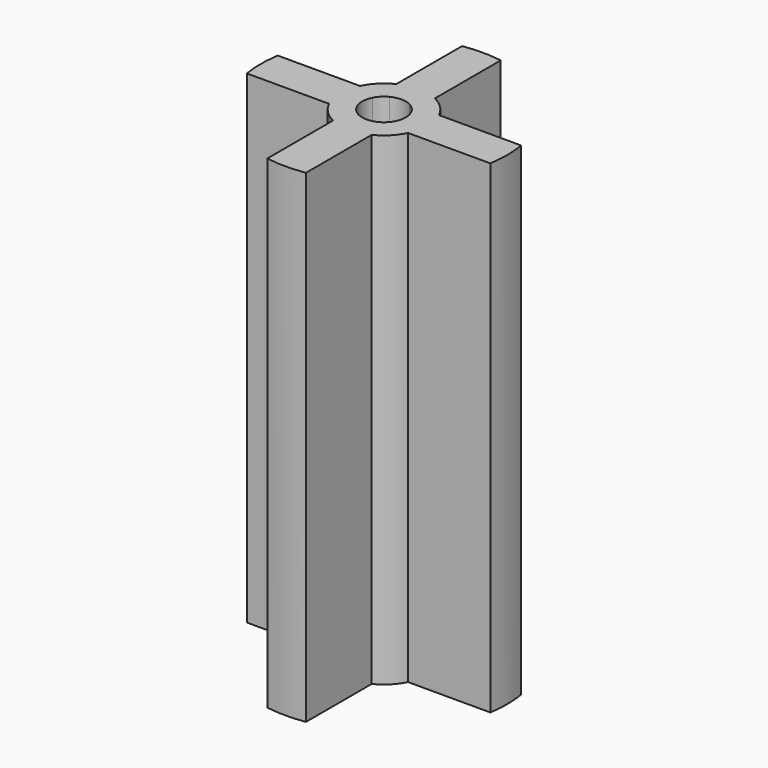
from build123d import *

# Parameters (mm, degrees)
F1_DEPTH = 84


# Not quite as in the source:
# - a pattern or mirror of a feature is missing from the dataset's text; its kind, count and spacing are read off the source's solid


with BuildPart() as f1:
    # F0 (on Top) → F1 (new body)
    with BuildSketch(Plane.XY):
        with BuildLine():
            ThreePointArc((-4, 12.4743737318), (0, 13.1), (4, 12.4743737318))
            Line((4, 12.4743737318), (4, 25.1843205189))
            Line((4, 25.1843205189), (-4, 25.1843205189))
            Line((-4, 25.1843205189), (-4, 12.4743737318))
        make_face()
        with BuildLine():
            Line((-4, 25.1843205189), (4, 25.1843205189))
            ThreePointArc((4, 25.1843205189), (0, 25.5), (-4, 25.1843205189))
        make_face()
        with BuildLine():
            ThreePointArc((25.5, 0), (25.4209576259, 2.0062186779), (25.1843205189, 4))
            Line((25.1843205189, 4), (25.1843205189, -4))
            ThreePointArc((25.1843205189, -4), (25.4209576259, -2.0062186779), (25.5, 0))
        make_face()
        with BuildLine():
            Line((25.1843205189, 4), (12.4743737318, 4))
            ThreePointArc((12.4743737318, 4), (12.942648413, 2.0243152069), (13.1, 0))
            ThreePointArc((13.1, 0), (12.942648413, -2.0243152069), (12.4743737318, -4))
            Line((12.4743737318, -4), (25.1843205189, -4))
            Line((25.1843205189, -4), (25.1843205189, 4))
        make_face()
        with BuildLine():
            ThreePointArc((-4, -25.1843205189), (0, -25.5), (4, -25.1843205189))
            Line((4, -25.1843205189), (-4, -25.1843205189))
        make_face()
        with BuildLine():
            Line((-25.1843205189, -4), (-25.1843205189, 4))
            ThreePointArc((-25.1843205189, 4), (-25.5, 0), (-25.1843205189, -4))
        make_face()
        with BuildLine():
            ThreePointArc((-12.4743737318, -4), (-13.1, 0), (-12.4743737318, 4))
            Line((-12.4743737318, 4), (-25.1843205189, 4))
            Line((-25.1843205189, 4), (-25.1843205189, -4))
            Line((-25.1843205189, -4), (-12.4743737318, -4))
        make_face()
        with BuildLine():
            Line((4, -25.1843205189), (4, -12.4743737318))
            ThreePointArc((4, -12.4743737318), (0, -13.1), (-4, -12.4743737318))
            Line((-4, -12.4743737318), (-4, -25.1843205189))
            Line((-4, -25.1843205189), (4, -25.1843205189))
        make_face()
        with BuildLine():
            Line((-8.1737384348, 4), (-10.3542261903, 4))
            ThreePointArc((-10.3542261903, 4), (-11.1, 0), (-10.3542261903, -4))
            Line((-10.3542261903, -4), (-8.1737384348, -4))
            ThreePointArc((-8.1737384348, -4), (-9.1, 0), (-8.1737384348, 4))
        make_face()
        with BuildLine():
            ThreePointArc((-10.3542261903, -4), (-11.1, 0), (-10.3542261903, 4))
            Line((-10.3542261903, 4), (-12.4743737318, 4))
            ThreePointArc((-12.4743737318, 4), (-13.1, 0), (-12.4743737318, -4))
            Line((-12.4743737318, -4), (-10.3542261903, -4))
        make_face()
        with BuildLine():
            Line((4, 8.1737384348), (4, 10.3542261903))
            ThreePointArc((4, 10.3542261903), (0, 11.1), (-4, 10.3542261903))
            Line((-4, 10.3542261903), (-4, 8.1737384348))
            ThreePointArc((-4, 8.1737384348), (0, 9.1), (4, 8.1737384348))
        make_face()
        with BuildLine():
            ThreePointArc((-4, 10.3542261903), (0, 11.1), (4, 10.3542261903))
            Line((4, 10.3542261903), (4, 12.4743737318))
            ThreePointArc((4, 12.4743737318), (0, 13.1), (-4, 12.4743737318))
            Line((-4, 12.4743737318), (-4, 10.3542261903))
        make_face()
        with BuildLine():
            ThreePointArc((10.3542261903, 4), (10.9119638634, 2.0344642154), (11.1, 0))
            ThreePointArc((11.1, 0), (10.9119638634, -2.0344642154), (10.3542261903, -4))
            Line((10.3542261903, -4), (12.4743737318, -4))
            ThreePointArc((12.4743737318, -4), (12.942648413, -2.0243152069), (13.1, 0))
            ThreePointArc((13.1, 0), (12.942648413, 2.0243152069), (12.4743737318, 4))
            Line((12.4743737318, 4), (10.3542261903, 4))
        make_face()
        with BuildLine():
            ThreePointArc((10.3542261903, -4), (10.9119638634, -2.0344642154), (11.1, 0))
            ThreePointArc((11.1, 0), (10.9119638634, 2.0344642154), (10.3542261903, 4))
            Line((10.3542261903, 4), (8.1737384348, 4))
            ThreePointArc((8.1737384348, 4), (8.8654108691, 2.052922337), (9.1, 0))
            ThreePointArc((9.1, 0), (8.8654108691, -2.052922337), (8.1737384348, -4))
            Line((8.1737384348, -4), (10.3542261903, -4))
        make_face()
        with BuildLine():
            ThreePointArc((-4, -10.3542261903), (0, -11.1), (4, -10.3542261903))
            Line((4, -10.3542261903), (4, -8.1737384348))
            ThreePointArc((4, -8.1737384348), (0, -9.1), (-4, -8.1737384348))
            Line((-4, -8.1737384348), (-4, -10.3542261903))
        make_face()
        with BuildLine():
            Line((4, -12.4743737318), (4, -10.3542261903))
            ThreePointArc((4, -10.3542261903), (0, -11.1), (-4, -10.3542261903))
            Line((-4, -10.3542261903), (-4, -12.4743737318))
            ThreePointArc((-4, -12.4743737318), (0, -13.1), (4, -12.4743737318))
        make_face()
        with BuildLine():
            Line((-4, 4), (-8.1737384348, 4))
            ThreePointArc((-8.1737384348, 4), (-9.1, 0), (-8.1737384348, -4))
            Line((-8.1737384348, -4), (-4, -4))
            Line((-4, -4), (-4, -2.0615528128))
            ThreePointArc((-4, -2.0615528128), (-4.5, 0), (-4, 2.0615528128))
            Line((-4, 2.0615528128), (-4, 4))
        make_face()
        with BuildLine():
            Line((-4, 4), (-4, 8.1737384348))
            ThreePointArc((-4, 8.1737384348), (-6.4346717088, 6.4346717088), (-8.1737384348, 4))
            Line((-8.1737384348, 4), (-4, 4))
        make_face()
        with BuildLine():
            Line((4, 4), (4, 8.1737384348))
            ThreePointArc((4, 8.1737384348), (0, 9.1), (-4, 8.1737384348))
            Line((-4, 8.1737384348), (-4, 4))
            Line((-4, 4), (-2.0615528128, 4))
            ThreePointArc((-2.0615528128, 4), (0, 4.5), (2.0615528128, 4))
            Line((2.0615528128, 4), (4, 4))
        make_face()
        with BuildLine():
            Line((4, 4), (8.1737384348, 4))
            ThreePointArc((8.1737384348, 4), (6.4346717088, 6.4346717088), (4, 8.1737384348))
            Line((4, 8.1737384348), (4, 4))
        make_face()
        with BuildLine():
            ThreePointArc((9.1, 0), (8.8654108691, 2.052922337), (8.1737384348, 4))
            Line((8.1737384348, 4), (4, 4))
            Line((4, 4), (4, 2.0615528128))
            ThreePointArc((4, 2.0615528128), (4.3732139211, 1.0606601718), (4.5, 0))
            ThreePointArc((4.5, 0), (4.3732139211, -1.0606601718), (4, -2.0615528128))
            Line((4, -2.0615528128), (4, -4))
            Line((4, -4), (8.1737384348, -4))
            ThreePointArc((8.1737384348, -4), (8.8654108691, -2.052922337), (9.1, 0))
        make_face()
        with BuildLine():
            ThreePointArc((-4, -8.1737384348), (0, -9.1), (4, -8.1737384348))
            Line((4, -8.1737384348), (4, -4))
            Line((4, -4), (2.0615528128, -4))
            ThreePointArc((2.0615528128, -4), (0, -4.5), (-2.0615528128, -4))
            Line((-2.0615528128, -4), (-4, -4))
            Line((-4, -4), (-4, -8.1737384348))
        make_face()
        with BuildLine():
            ThreePointArc((-8.1737384348, -4), (-6.4346717088, -6.4346717088), (-4, -8.1737384348))
            Line((-4, -8.1737384348), (-4, -4))
            Line((-4, -4), (-8.1737384348, -4))
        make_face()
        with BuildLine():
            ThreePointArc((4, -8.1737384348), (6.4346717088, -6.4346717088), (8.1737384348, -4))
            Line((8.1737384348, -4), (4, -4))
            Line((4, -4), (4, -8.1737384348))
        make_face()
        with BuildLine():
            Line((2.0615528128, -4), (4, -4))
            Line((4, -4), (4, -2.0615528128))
            ThreePointArc((4, -2.0615528128), (3.1819805153, -3.1819805153), (2.0615528128, -4))
        make_face()
        with BuildLine():
            Line((-4, -2.0615528128), (-4, -4))
            Line((-4, -4), (-2.0615528128, -4))
            ThreePointArc((-2.0615528128, -4), (-3.1819805153, -3.1819805153), (-4, -2.0615528128))
        make_face()
        with BuildLine():
            Line((-2.0615528128, 4), (-4, 4))
            Line((-4, 4), (-4, 2.0615528128))
            ThreePointArc((-4, 2.0615528128), (-3.1819805153, 3.1819805153), (-2.0615528128, 4))
        make_face()
        with BuildLine():
            Line((4, 2.0615528128), (4, 4))
            Line((4, 4), (2.0615528128, 4))
            ThreePointArc((2.0615528128, 4), (3.1819805153, 3.1819805153), (4, 2.0615528128))
        make_face()
    extrude(amount=-F1_DEPTH)

    # F1_copies: F1 across plane


with BuildPart() as f1_1:
    add(f1.part)
    add(f1.part.mirror(Plane(origin=(0, 0, -50), x_dir=(-1, 0, 0), z_dir=(0, 0, -1))))


solid = f1_1.part
